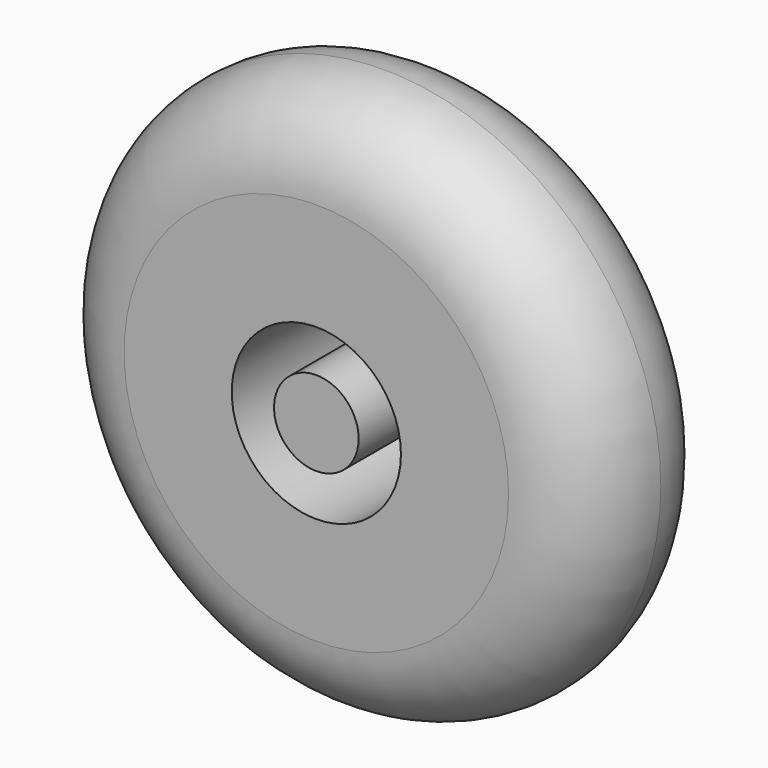
from build123d import *

# Parameters (mm, degrees)
F0_R     = 5.5
F1_DEPTH = 22
F0_R_2   = 36
F0_R_3   = 11
F2_R     = 11
F3_R     = 10.99999


# Not quite as in the source:
# - a fillet or chamfer is up to 0.001 mm smaller than in the source, because OpenCascade refuses the exact size


with BuildPart() as f1:
    # F0 (on Front) → F1 (new body)
    with BuildSketch(Plane.XZ):
        Circle(F0_R)
    extrude(amount=F1_DEPTH)


with BuildPart() as f1b:
    # F0 (on Front) → F1, piece 2 (new body)
    with BuildSketch(Plane.XZ):
        Circle(F0_R_2)
        Circle(F0_R_3, mode=Mode.SUBTRACT)
    extrude(amount=F1_DEPTH)

    # F2
    f2_edges = [f1b.edges().sort_by_distance(p)[0] for p in [
        (-36, -22, 0),
    ]]
    fillet(f2_edges, radius=F2_R)

    # F3 (radius 11 in the source; OpenCascade refuses exactly that, so slightly less here)
    f3_edges = [f1b.edges().sort_by_distance(p)[0] for p in [
        (-36, 0, 0),
    ]]
    fillet(f3_edges, radius=F3_R)


solid = Compound([f1.part, f1b.part])
